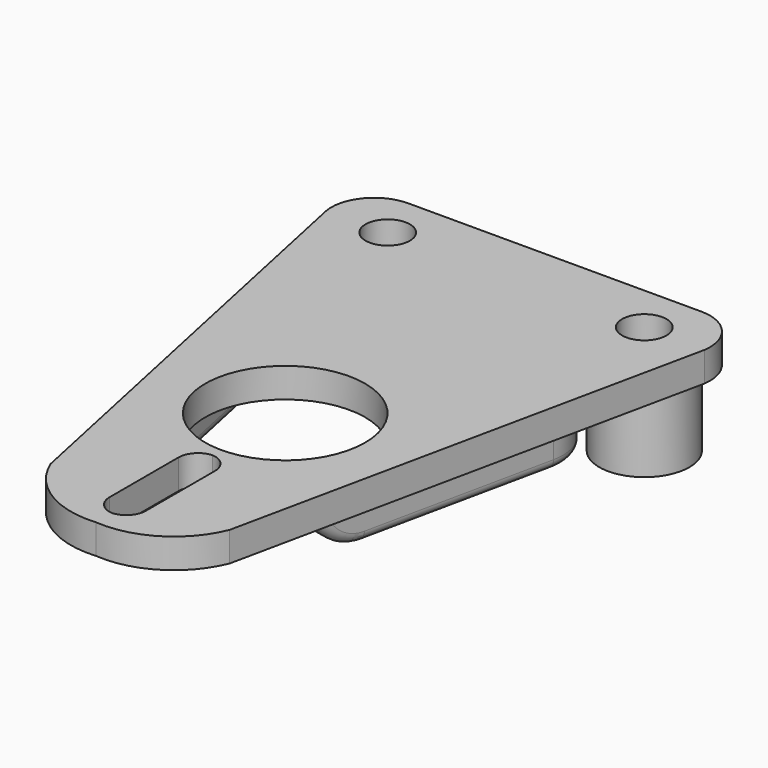
from build123d import *

# Parameters (mm, degrees)
F0_W        = 3.7012519315
F0_H        = 12.7320559695
F0_R        = 8.100129487
F0_R_2      = 2.25
F1_DEPTH    = 3
F2_T1_DEPTH = 3
F3_R        = 4.5649895604
F3_R_2      = 2.4116141927
F3_R_3      = 2.2420485947
F4_DEPTH    = 8
F6_DEPTH    = 3
F7_T1_DEPTH = 14.95289459
F7_T3_DEPTH = 26.4498235383
F7_T5_DEPTH = 26.4498235383
F8_R        = 1


# Not quite as in the source:
# - a fillet or chamfer that OpenCascade refuses, or shapes differently, is made with other operations: its cross-section is extruded or revolved along the edge and cut away or added


with BuildPart() as f1:
    # F0 (on Top) → F1 (new body)
    with BuildSketch(Plane.XY):
        with BuildLine():
            Line((14.8444259539, 34.1621562839), (0, 34.1621562839))
            Line((0, 34.1621562839), (-14.8444259539, 34.1621562839))
            ThreePointArc((-14.8444259539, 34.1621562839), (-18.1303110964, 32.6596806941), (-19.1433615983, 29.1915107518))
            Line((-19.1433615983, 29.1915107518), (-9.0677291155, -18.3654725552))
            ThreePointArc((-9.0677291155, -18.3654725552), (-5.4543132889, -22.6555173257), (0, -23.9638462663))
            ThreePointArc((0, -23.9638462663), (5.4543132889, -22.6555173257), (9.0677291155, -18.3654725552))
            Line((9.0677291155, -18.3654725552), (19.1433615983, 29.1915107518))
            ThreePointArc((19.1433615983, 29.1915107518), (18.1303110964, 32.6596806941), (14.8444259539, 34.1621562839))
        make_face()
        with Locations((0, -15.5778131448)):
            Rectangle(F0_W, F0_H, mode=Mode.SUBTRACT)
        Circle(F0_R, mode=Mode.SUBTRACT)
        with Locations((-13, 29.2403830344)):
            Circle(F0_R_2, mode=Mode.SUBTRACT)
        with Locations((13, 29.2403830344)):
            Circle(F0_R_2, mode=Mode.SUBTRACT)
    extrude(amount=F1_DEPTH)

    # F2: fillet of radius 2 on 4 edges, made by hand

    # F2_s2 → F2_t1 (join)
    with BuildSketch(Plane.XY):
        with BuildLine():
            ThreePointArc((0.1493740343, -9.21178516), (-1.2648395281, -9.7975715976), (-1.8506259657, -11.21178516))
            Line((-1.8506259657, -11.21178516), (-1.8506259657, -9.21178516))
            Line((-1.8506259657, -9.21178516), (0.1493740343, -9.21178516))
        make_face()
        with BuildLine():
            ThreePointArc((1.8506259657, -11.21178516), (1.2648395281, -9.7975715976), (-0.1493740343, -9.21178516))
            Line((-0.1493740343, -9.21178516), (1.8506259657, -9.21178516))
            Line((1.8506259657, -9.21178516), (1.8506259657, -11.21178516))
        make_face()
        with BuildLine():
            ThreePointArc((-1.8506259657, -19.9438411295), (-1.2648395281, -21.3580546919), (0.1493740343, -21.9438411295))
            Line((0.1493740343, -21.9438411295), (-1.8506259657, -21.9438411295))
            Line((-1.8506259657, -21.9438411295), (-1.8506259657, -19.9438411295))
        make_face()
        with BuildLine():
            ThreePointArc((1.8506259657, -19.9438411295), (1.2648395281, -21.3580546919), (-0.1493740343, -21.9438411295))
            Line((-0.1493740343, -21.9438411295), (1.8506259657, -21.9438411295))
            Line((1.8506259657, -21.9438411295), (1.8506259657, -19.9438411295))
        make_face()
    extrude(amount=F2_T1_DEPTH)

    # F3 (on face) → F4 (join)
    with BuildSketch(Plane(origin=(0, 0, 0), x_dir=(1, 0, 0), z_dir=(0, 0, -1))):
        with Locations((13, -29.2403830344)):
            Circle(F3_R)
        with Locations((13, -29.2403830344)):
            Circle(F3_R_2, mode=Mode.SUBTRACT)
        with Locations((-13, -29.2403830344)):
            Circle(F3_R)
        with Locations((-13, -29.2403830344)):
            Circle(F3_R_3, mode=Mode.SUBTRACT)
    extrude(amount=F4_DEPTH)

    # F5 (on face) → F6 (join)
    with BuildSketch(Plane(origin=(0, 0, 0), x_dir=(1, 0, 0), z_dir=(0, 0, -1))):
        Polygon((-7.118105705, 8.1281888095), (-10.5773922314, 8.8652892849), (-16.5612712118, -19.2176554765), (-13.1019846854, -19.9547559519), align=None)
        Polygon((16.5612712118, -19.2176554765), (10.5773922314, 8.8652892849), (7.118105705, 8.1281888095), (13.1019846854, -19.9547559519), align=None)
    extrude(amount=F6_DEPTH)

    # F7: fillet of radius 5 on 4 edges, made by hand

    # F7_s2 → F7_t1 (cut)
    with BuildSketch(Plane.XY.offset(-14.95289459)):
        with BuildLine():
            ThreePointArc((-13.1019846854, 19.9547559519), (-15.2257590624, 17.6540998095), (-15.5648763993, 14.5414745957))
            Line((-15.5648763993, 14.5414745957), (-16.5612712118, 19.2176554765))
            Line((-16.5612712118, 19.2176554765), (-13.1019846854, 19.9547559519))
        make_face()
        with BuildLine():
            ThreePointArc((15.5648763993, 14.5414745957), (15.2257590624, 17.6540998095), (13.1019846854, 19.9547559519))
            Line((13.1019846854, 19.9547559519), (16.5612712118, 19.2176554765))
            Line((16.5612712118, 19.2176554765), (15.5648763993, 14.5414745957))
        make_face()
    extrude(amount=F7_T1_DEPTH, mode=Mode.SUBTRACT)

    # F7_s4 → F7_t3 (cut)
    with BuildSketch(Plane(origin=(23.1298700172, -4.9284839674, 0), x_dir=(0, 0, 1), z_dir=(-0.9780436123, 0.2084003178, 0))):
        with BuildLine():
            ThreePointArc((0, -6.4663076535), (-2.1833001327, -4.622344746), (-3, -1.8837319585))
            Line((-3, -1.8837319585), (-3, -6.4663076535))
            Line((-3, -6.4663076535), (0, -6.4663076535))
        make_face()
    extrude(amount=F7_T3_DEPTH, mode=Mode.SUBTRACT)

    # F7_s6 → F7_t5 (cut)
    with BuildSketch(Plane(origin=(2.7392109406, 0.5836676641, 0), x_dir=(0, 0, 1), z_dir=(-0.9780436123, -0.2084003178, 0))):
        with BuildLine():
            ThreePointArc((0, -6.4663076535), (-2.1833001327, -4.622344746), (-3, -1.8837319585))
            Line((-3, -1.8837319585), (-3, -6.4663076535))
            Line((-3, -6.4663076535), (0, -6.4663076535))
        make_face()
    extrude(amount=F7_T5_DEPTH, mode=Mode.SUBTRACT)

    # F8
    f8_edges = [f1.edges().sort_by_distance(p)[0] for p in [
        (-10.58755, 8.154263, -3),
        (10.58755, 8.154263, -3),
        (13.548639, 5.079072, -3),
        (-13.548639, 5.079072, -3),
        (-15.225759, 17.6541, -3),
        (-10.961675, -7.061813, -2.1833),
        (-7.502388, -6.324713, -2.1833),
        (15.225759, 17.6541, -3),
        (7.502388, -6.324713, -2.1833),
        (10.961675, -7.061813, -2.1833),
    ]]
    fillet(f8_edges, radius=F8_R)


solid = f1.part
